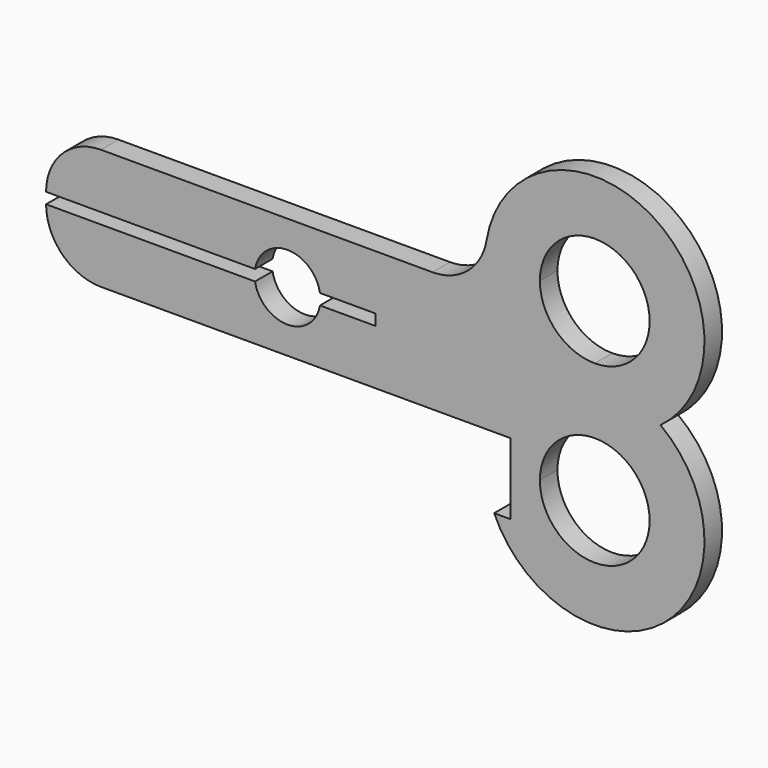
from build123d import *

# Parameters (mm, degrees)
F1_DEPTH = 2
F2_R     = 5
F4_DEPTH = 2
F6_DEPTH = 25


# Not quite as in the source:
# - a feature names something its author has since deleted; it is built from what else it names


with BuildPart() as f1:
    # F0 (on Front) → F1 (new body)
    with BuildSketch(Plane.XZ):
        with BuildLine():
            Line((0, 5.5), (0, 0))
            Line((0, 0), (40, 0))
            Line((40, 0), (40, 5.5))
            Line((40, 5.5), (25, 5.5))
            ThreePointArc((25, 5.5), (22, 2.5), (19, 5.5))
            Line((19, 5.5), (0, 5.5))
        make_face()
        with BuildLine():
            Line((40, 5.5), (40, 0))
            Line((40, 0), (40, -2.5))
            ThreePointArc((40, -2.5), (41.05572809, 1.972135955), (44, 5.5))
            Line((44, 5.5), (40, 5.5))
        make_face()
        with BuildLine():
            Line((0, 11), (0, 5.5))
            Line((0, 5.5), (19, 5.5))
            ThreePointArc((19, 5.5), (22, 8.5), (25, 5.5))
            Line((25, 5.5), (40, 5.5))
            Line((40, 5.5), (40, 11))
            Line((40, 11), (0, 11))
        make_face()
        with BuildLine():
            Line((40, 11), (40, 5.5))
            Line((40, 5.5), (44, 5.5))
            ThreePointArc((44, 5.5), (41.05572809, 9.027864045), (40, 13.5))
            Line((40, 13.5), (40, 11))
        make_face()
        with BuildLine():
            Line((45, -2.5), (40, -2.5))
            ThreePointArc((40, -2.5), (50, -12.5), (60, -2.5))
            ThreePointArc((60, -2.5), (58.94427191, 1.972135955), (56, 5.5))
            ThreePointArc((56, 5.5), (53.1622776602, 4.0131670195), (50, 3.5))
            Line((50, 3.5), (50, 2.5))
            ThreePointArc((50, 2.5), (53.5355339059, 1.0355339059), (55, -2.5))
            ThreePointArc((55, -2.5), (50, -7.5), (45, -2.5))
        make_face()
        with BuildLine():
            ThreePointArc((44, 5.5), (41.05572809, 1.972135955), (40, -2.5))
            Line((40, -2.5), (45, -2.5))
            ThreePointArc((45, -2.5), (46.4644660941, 1.0355339059), (50, 2.5))
            Line((50, 2.5), (50, 3.5))
            ThreePointArc((50, 3.5), (46.8377223398, 4.0131670195), (44, 5.5))
        make_face()
        with BuildLine():
            ThreePointArc((40, 13.5), (41.05572809, 9.027864045), (44, 5.5))
            ThreePointArc((44, 5.5), (46.8377223398, 6.9868329805), (50, 7.5))
            Line((50, 7.5), (50, 8.5))
            ThreePointArc((50, 8.5), (46.4644660941, 9.9644660941), (45, 13.5))
            Line((45, 13.5), (40, 13.5))
        make_face()
        with BuildLine():
            Line((50, 5.5), (44, 5.5))
            ThreePointArc((44, 5.5), (46.8377223398, 4.0131670195), (50, 3.5))
            Line((50, 3.5), (50, 5.5))
        make_face()
        with BuildLine():
            ThreePointArc((50, 7.5), (46.8377223398, 6.9868329805), (44, 5.5))
            Line((44, 5.5), (50, 5.5))
            Line((50, 5.5), (50, 7.5))
        make_face()
        with BuildLine():
            ThreePointArc((60, 13.5), (50, 23.5), (40, 13.5))
            Line((40, 13.5), (45, 13.5))
            ThreePointArc((45, 13.5), (50, 18.5), (55, 13.5))
            ThreePointArc((55, 13.5), (53.5355339059, 9.9644660941), (50, 8.5))
            Line((50, 8.5), (50, 7.5))
            ThreePointArc((50, 7.5), (53.1622776602, 6.9868329805), (56, 5.5))
            ThreePointArc((56, 5.5), (58.94427191, 9.027864045), (60, 13.5))
        make_face()
        with BuildLine():
            ThreePointArc((56, 5.5), (53.1622776602, 6.9868329805), (50, 7.5))
            Line((50, 7.5), (50, 5.5))
            Line((50, 5.5), (56, 5.5))
        make_face()
        with BuildLine():
            Line((50, 5.5), (50, 3.5))
            ThreePointArc((50, 3.5), (53.1622776602, 4.0131670195), (56, 5.5))
            Line((56, 5.5), (50, 5.5))
        make_face()
    extrude(amount=F1_DEPTH)

    # F2
    f2_edges = [f1.edges().sort_by_distance(p)[0] for p in [
        (40, -1, 11),
        (0, -1, 11),
        (0, -1, 0),
    ]]
    fillet(f2_edges, radius=F2_R)

    # F3 (on face) → F4 (cut, through all)
    with BuildSketch(Plane.XZ.offset(2)):
        with BuildLine():
            Line((19.0419601085, 6), (0, 6))
            Line((0, 6), (0, 5))
            Line((0, 5), (19.0419601085, 5))
            ThreePointArc((19.0419601085, 5), (19, 5.5), (19.0419601085, 6))
        make_face()
        with BuildLine():
            Line((30, 6), (24.9580398915, 6))
            ThreePointArc((24.9580398915, 6), (24.9894915684, 5.7508787808), (25, 5.5))
            ThreePointArc((25, 5.5), (24.9894915684, 5.2491212192), (24.9580398915, 5))
            Line((24.9580398915, 5), (30, 5))
            Line((30, 5), (30, 6))
        make_face()
    extrude(amount=-F4_DEPTH, mode=Mode.SUBTRACT)

    # F5 (on face) → F6 (cut)
    with BuildSketch(Plane.XZ.offset(2)):
        with BuildLine():
            ThreePointArc((40, -2.5), (40.2109368707, -4.5430964369), (40.8348486101, -6.5))
            Line((40.8348486101, -6.5), (42.3348486101, -6.5))
            Line((42.3348486101, -6.5), (42.3348486101, 0))
            Line((42.3348486101, 0), (40.3175416345, 0))
            ThreePointArc((40.3175416345, 0), (40.0797030373, -1.2399570752), (40, -2.5))
        make_face()
        with BuildLine():
            ThreePointArc((40, -2.5), (40.0797030373, -1.2399570752), (40.3175416345, 0))
            Line((40.3175416345, 0), (40, 0))
            Line((40, 0), (40, -2.5))
        make_face()
    extrude(amount=-F6_DEPTH, mode=Mode.SUBTRACT)


solid = f1.part
